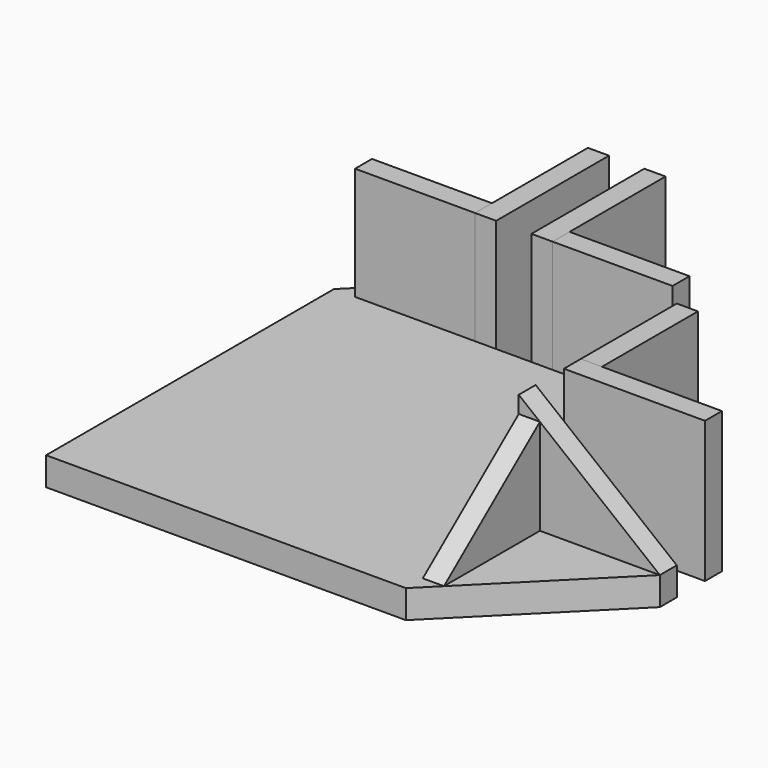
from build123d import *

# Parameters (mm, degrees)
F1_DEPTH = 4
F2_W     = 3
F2_H     = 17
F3_DEPTH = 20
F2_W_2   = 17
F2_H_2   = 3
F4_DEPTH = 20
F6_DEPTH = 3
F8_DEPTH = 3


with BuildPart() as f1:
    # F0 (on Top) → F1 (new body)
    with BuildSketch(Plane.XY):
        Polygon((-25.5, -25.5), (25.5, -25.5), (25.5, -5.5), (25.5, 5.5), (25.5, 25.5), (5.5, 25.5), (-5.5, 25.5), (-25.5, 25.5), align=None)
        Polygon((25.5, -5.5), (25.5, -25.5), (45.5, -5.5), align=None)
        Polygon((-5.5, 45.5), (-25.5, 25.5), (-5.5, 25.5), align=None)
        Polygon((25.5, 25.5), (25.5, 5.5), (45.5, 5.5), align=None)
        Polygon((5.5, 25.5), (25.5, 25.5), (5.5, 45.5), align=None)
    extrude(amount=F1_DEPTH)


with BuildPart() as f3:
    # F2 (on Top) → F3 (new body)
    with BuildSketch(Plane.XY):
        with Locations((27, -14)):
            Rectangle(F2_W, F2_H)
    extrude(amount=F3_DEPTH)

    # F5 (on face) → F6 (cut, through all)
    with BuildSketch(Plane(origin=(25.5, 0, 0), x_dir=(0, -1, 0), z_dir=(-1, 0, 0))):
        Polygon((5.5, 20), (5.5, 17.6), (22.5, 4), (22.5, 20), align=None)
    extrude(amount=-F6_DEPTH, mode=Mode.SUBTRACT)


with BuildPart() as f3b:
    # F2 (on Top) → F3, piece 2 (new body)
    with BuildSketch(Plane.XY):
        with Locations((27, 14)):
            Rectangle(F2_W, F2_H)
    extrude(amount=F3_DEPTH)


with BuildPart() as f3c:
    # F2 (on Top) → F3, piece 3 (new body)
    with BuildSketch(Plane.XY):
        with Locations((14, 27)):
            Rectangle(F2_W_2, F2_H_2)
    extrude(amount=F3_DEPTH)


with BuildPart() as f3d:
    # F2 (on Top) → F3, piece 4 (new body)
    with BuildSketch(Plane.XY):
        with Locations((-14, 27)):
            Rectangle(F2_W_2, F2_H_2)
    extrude(amount=F3_DEPTH)


with BuildPart() as f4:
    # F2 (on Top) → F4 (new body)
    with BuildSketch(Plane.XY):
        Polygon((28.5, 5.5), (25.5, 5.5), (25.5, 2.5), (45.5, 2.5), (45.5, 5.5), align=None)
    extrude(amount=F4_DEPTH)


with BuildPart() as f4b:
    # F2 (on Top) → F4, piece 2 (new body)
    with BuildSketch(Plane.XY):
        Polygon((45.5, -2.5), (25.5, -2.5), (25.5, -5.5), (28.5, -5.5), (45.5, -5.5), align=None)
    extrude(amount=F4_DEPTH)

    # F7 (on face) → F8 (cut, through all)
    with BuildSketch(Plane.XZ.offset(5.5)):
        Polygon((45.5, 20), (25.5, 20), (45.5, 4), align=None)
    extrude(amount=-F8_DEPTH, mode=Mode.SUBTRACT)


with BuildPart() as f4c:
    # F2 (on Top) → F4, piece 3 (new body)
    with BuildSketch(Plane.XY):
        Polygon((2.5, 45.5), (2.5, 25.5), (5.5, 25.5), (5.5, 28.5), (5.5, 45.5), align=None)
    extrude(amount=F4_DEPTH)


with BuildPart() as f4d:
    # F2 (on Top) → F4, piece 4 (new body)
    with BuildSketch(Plane.XY):
        Polygon((-5.5, 28.5), (-5.5, 25.5), (-2.5, 25.5), (-2.5, 45.5), (-5.5, 45.5), align=None)
    extrude(amount=F4_DEPTH)


solid = Compound([f1.part, f3.part, f3b.part, f3c.part, f3d.part, f4.part, f4b.part, f4c.part, f4d.part])
